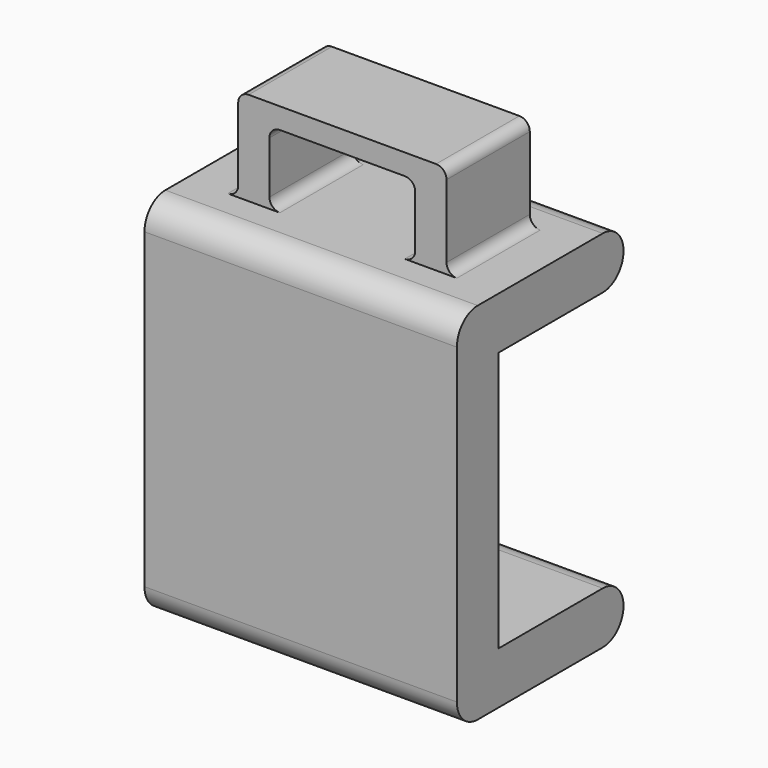
from build123d import *

# Parameters (mm, degrees)
F1_DEPTH = 15
F2_W     = 20
F2_H     = 10
F3_DEPTH = 9
F4_R     = 2.49999
F5_W     = 14
F5_H     = 7
F6_DEPTH = 10
F7_R     = 1


# Not quite as in the source:
# - a fillet or chamfer is up to 0.001 mm smaller than in the source, because OpenCascade refuses the exact size


with BuildPart() as f1:
    # F0 (on Right) → F1 (new body, symmetric)
    with BuildSketch(Plane.YZ):
        Polygon((15, 12.5), (15, 17.5), (-5, 17.5), (-5, -17.5), (15, -17.5), (15, -12.5), (0, -12.5), (0, 12.5), align=None)
    extrude(amount=F1_DEPTH, both=True)

    # F2 (on face) → F3 (join)
    with BuildSketch(Plane.XY.offset(17.5)):
        with Locations((0, 5)):
            Rectangle(F2_W, F2_H)
    extrude(amount=F3_DEPTH)

    # F4 (radius 2.5 in the source; OpenCascade refuses exactly that, so slightly less here)
    f4_edges = [f1.edges().sort_by_distance(p)[0] for p in [
        (0, 15, 12.5),
        (0, 15, -12.5),
        (0, 15, 17.5),
        (0, 15, -17.5),
        (0, -5, 17.5),
        (0, -5, -17.5),
    ]]
    fillet(f4_edges, radius=F4_R)

    # F5 (on face) → F6 (cut, through all)
    with BuildSketch(Plane.XZ):
        with Locations((0, 21)):
            Rectangle(F5_W, F5_H)
    extrude(amount=-F6_DEPTH, mode=Mode.SUBTRACT)

    # F7
    f7_edges = [f1.edges().sort_by_distance(p)[0] for p in [
        (-7, 5, 17.5),
        (-7, 5, 24.5),
        (7, 5, 17.5),
        (7, 5, 24.5),
        (-10, 5, 17.5),
        (-10, 5, 26.5),
        (10, 5, 26.5),
        (10, 5, 17.5),
    ]]
    fillet(f7_edges, radius=F7_R)


solid = f1.part
